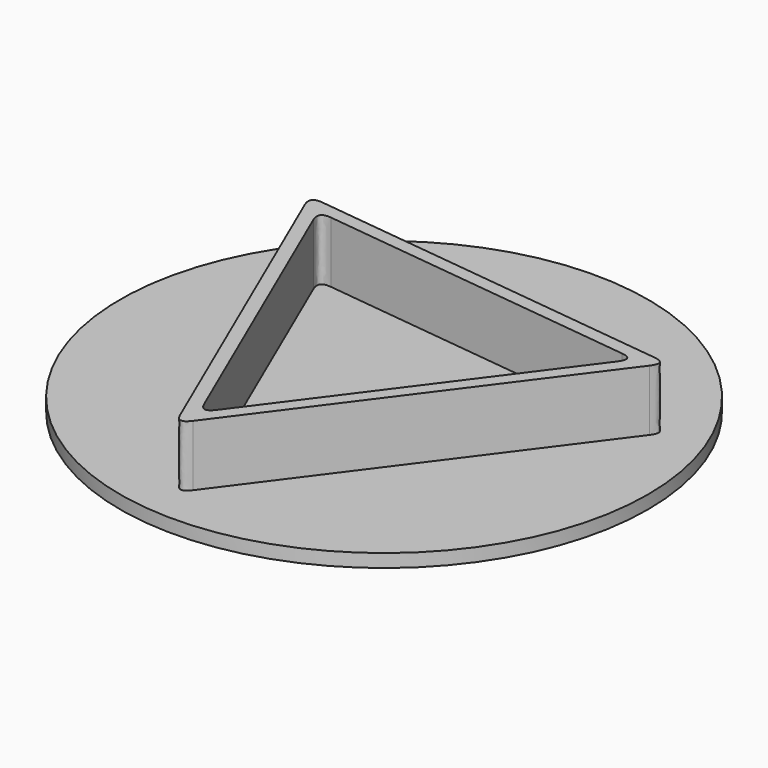
from build123d import *

# Parameters (mm, degrees)
F0_R        = 32
F1_DEPTH    = 1.6
F2_DEPTH    = 1.6
F3_DEPTH    = 9
F4_T1_DEPTH = 7.4
F4_T3_DEPTH = 11.7301270189


# Not quite as in the source:
# - a fillet or chamfer that OpenCascade refuses, or shapes differently, is made with other operations: its cross-section is extruded or revolved along the edge and cut away or added


with BuildPart() as f1:
    # F0 (on Top) → F1 (new body)
    with BuildSketch(Plane.XY):
        Circle(F0_R)
        Polygon((-3.2203362492, -27.6128490823), (-22.3032606516, 16.5953175417), (25.5235969007, 11.0175315406), align=None, mode=Mode.SUBTRACT)
        Polygon((25.5235969007, 11.0175315406), (-22.3032606516, 16.5953175417), (-3.2203362492, -27.6128490823), align=None)
        Polygon((-2.8496500622, -24.434391634), (-19.7359788499, 14.6850651628), (22.5856289122, 9.7493264712), align=None, mode=Mode.SUBTRACT)
    extrude(amount=F1_DEPTH)

    # F0 (on Top) → F2 (join)
    with BuildSketch(Plane.XY):
        Polygon((22.5856289122, 9.7493264712), (-19.7359788499, 14.6850651628), (-2.8496500622, -24.434391634), align=None)
    extrude(amount=F2_DEPTH)

    # F0 (on Top) → F3 (join)
    with BuildSketch(Plane.XY):
        Polygon((25.5235969007, 11.0175315406), (-22.3032606516, 16.5953175417), (-3.2203362492, -27.6128490823), align=None)
        Polygon((-2.8496500622, -24.434391634), (-19.7359788499, 14.6850651628), (22.5856289122, 9.7493264712), align=None, mode=Mode.SUBTRACT)
    extrude(amount=F3_DEPTH)

    # F4: fillet of radius 1 on 6 edges, made by hand

    # F4_s2 → F4_t1 (join)
    with BuildSketch(Plane.XY.offset(1.6)):
        with BuildLine():
            add(Edge.make_bspline(
                [(-3.5360861918, -22.844169813), (-2.8496500622, -24.434391634), (-1.8156956324, -23.0448095972)],
                knots=[0, 0, 0, 1, 1, 1], degree=2, weights=[1, 1, 1]))
            Line((-1.8156956324, -23.0448095972), (-2.8496500622, -24.434391634))
            Line((-2.8496500622, -24.434391634), (-3.5360861918, -22.844169813))
        make_face()
        with BuildLine():
            add(Edge.make_bspline(
                [(20.8652383527, 9.9499662554), (22.5856289122, 9.7493264712), (21.5516744823, 8.3597444344)],
                knots=[0, 0, 0, 1, 1, 1], degree=2, weights=[1, 1, 1]))
            Line((21.5516744823, 8.3597444344), (22.5856289122, 9.7493264712))
            Line((22.5856289122, 9.7493264712), (20.8652383527, 9.9499662554))
        make_face()
        with BuildLine():
            add(Edge.make_bspline(
                [(-19.0495427204, 13.0948433418), (-19.7359788499, 14.6850651628), (-18.0155882905, 14.4844253786)],
                knots=[0, 0, 0, 1, 1, 1], degree=2, weights=[1, 1, 1]))
            Line((-18.0155882905, 14.4844253786), (-19.7359788499, 14.6850651628))
            Line((-19.7359788499, 14.6850651628), (-19.0495427204, 13.0948433418))
        make_face()
    extrude(amount=F4_T1_DEPTH)

    # F4_s4 → F4_t3 (cut)
    with BuildSketch(Plane.XY.offset(1.6)):
        with BuildLine():
            add(Edge.make_bspline(
                [(-3.9067723788, -26.0226272613), (-3.2203362492, -27.6128490823), (-2.1863818193, -26.2232670455)],
                knots=[0, 0, 0, 1, 1, 1], degree=2, weights=[1, 1, 1]))
            Line((-2.1863818193, -26.2232670455), (-3.2203362492, -27.6128490823))
            Line((-3.2203362492, -27.6128490823), (-3.9067723788, -26.0226272613))
        make_face()
        with BuildLine():
            add(Edge.make_bspline(
                [(23.8032063413, 11.2181713248), (25.5235969007, 11.0175315406), (24.4896424709, 9.6279495038)],
                knots=[0, 0, 0, 1, 1, 1], degree=2, weights=[1, 1, 1]))
            Line((24.4896424709, 9.6279495038), (25.5235969007, 11.0175315406))
            Line((25.5235969007, 11.0175315406), (23.8032063413, 11.2181713248))
        make_face()
        with BuildLine():
            add(Edge.make_bspline(
                [(-20.5828700921, 16.3946777575), (-22.3032606516, 16.5953175417), (-21.616824522, 15.0050957207)],
                knots=[0, 0, 0, 1, 1, 1], degree=2, weights=[1, 1, 1]))
            Line((-21.616824522, 15.0050957207), (-22.3032606516, 16.5953175417))
            Line((-22.3032606516, 16.5953175417), (-20.5828700921, 16.3946777575))
        make_face()
    extrude(amount=F4_T3_DEPTH, mode=Mode.SUBTRACT)


solid = f1.part
